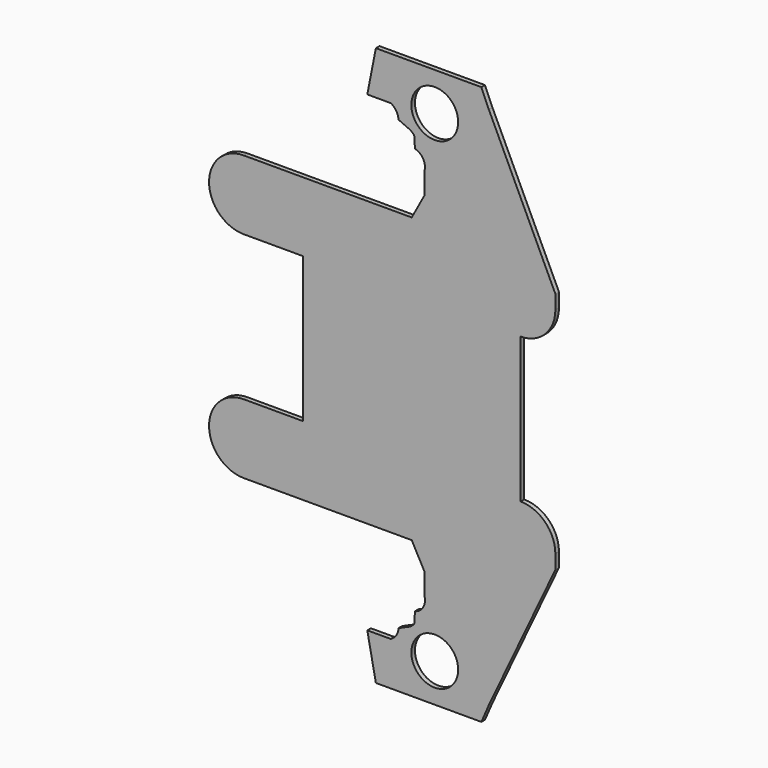
from build123d import *

# Parameters (mm, degrees)
F0_R     = 16.51
F1_DEPTH = 3.175


# Not quite as in the source:
# - ends of sketch curves that miss each other by under 0.0002 mm in the source are joined
# - a feature names something its author has since deleted; it is built from what else it names


with BuildPart() as f1:
    # F0 (on Front) → F1 (new body)
    with BuildSketch(Plane.XZ):
        with BuildLine():
            Line((72.172606051, -154.628444229), (72.172606051, -76.840944229))
            Line((72.172606051, -76.840944229), (72.172606051, -64.494198626))
            ThreePointArc((72.172606051, -64.494198626), (89.5045003647, -57.3150929397), (96.683606051, -39.983198626))
            Line((96.683606051, -39.983198626), (96.683606051, -30.0584486086))
            Line((96.683606051, -30.0584486086), (49.8026024117, 69.0988139849))
            Line((49.8026024117, 69.0988139849), (44.4719158113, 81.3992435336))
            Line((44.4719158113, 81.3992435336), (-29.9480052508, 81.3992435336))
            Line((-29.9480052508, 81.3992435336), (-35.9978974571, 50.6829957967))
            Line((-35.9978974571, 50.6829957967), (-19.4879078689, 50.6714224456))
            ThreePointArc((-19.4879078689, 50.6714224456), (-15.5812211009, 47.1637298884), (-13.9720730804, 42.1660573792))
            Line((-13.9720730804, 42.1660573792), (-5.4024819992, 38.3506346508))
            Line((-5.4024819992, 38.3506346508), (-2.9009456417, 36.1038269705))
            Line((-2.9009456417, 36.1038269705), (-2.3647786124, 27.9011076368))
            ThreePointArc((-2.3647786124, 27.9011076368), (3.4353485173, 23.5426794776), (4.3712937617, 16.3481414632))
            Line((4.3712937617, 16.3481414632), (4.2880811809, 16.2515226396))
            Line((4.2880811809, 16.2515226396), (4.2880776677, 1.0115236557))
            Line((4.2880776677, 1.0115236557), (-4.6405893252, -15.5276898319))
            Line((-4.6405893252, -15.5276898319), (-123.1544493252, -15.5276898319))
            ThreePointArc((-123.1544493252, -15.5276898319), (-147.6377037222, -40.010944229), (-123.1544493252, -64.494198626))
            Line((-123.1544493252, -64.494198626), (-81.4537847014, -64.494198626))
            Line((-81.4537847014, -64.494198626), (-81.4537847014, -76.840944229))
            Line((-81.4537847014, -76.840944229), (-81.4537847014, -154.628444229))
            Line((-81.4537847014, -154.628444229), (-81.4537847014, -166.9751898319))
            Line((-81.4537847014, -166.9751898319), (-123.1544493252, -166.9751898319))
            ThreePointArc((-123.1544493252, -166.9751898319), (-147.6377037222, -191.458444229), (-123.1544493252, -215.941698626))
            Line((-123.1544493252, -215.941698626), (-4.6405893252, -215.941698626))
            Line((-4.6405893252, -215.941698626), (4.2880776677, -232.4809121137))
            Line((4.2880776677, -232.4809121137), (4.2880811809, -247.7209110976))
            Line((4.2880811809, -247.7209110976), (4.3712937617, -247.8175299212))
            ThreePointArc((4.3712937617, -247.8175299212), (3.4353485173, -255.0120679356), (-2.3647786124, -259.3704960948))
            Line((-2.3647786124, -259.3704960948), (-2.9009456417, -267.5732154285))
            Line((-2.9009456417, -267.5732154285), (-5.4024819992, -269.8200231088))
            Line((-5.4024819992, -269.8200231088), (-13.9720735102, -273.6354510709))
            ThreePointArc((-13.9720735102, -273.6354510709), (-15.5812211009, -278.6331183464), (-19.487905219, -282.1408109018))
            Line((-19.487905219, -282.1408109018), (-35.9978974571, -282.1523842547))
            Line((-35.9978974571, -282.1523842547), (-29.9480052508, -312.8686319916))
            Line((-29.9480052508, -312.8686319916), (44.4719158113, -312.8686319916))
            Line((44.4719158113, -312.8686319916), (49.8026024117, -300.5682024429))
            Line((49.8026024117, -300.5682024429), (96.683606051, -201.4109398494))
            Line((96.683606051, -201.4109398494), (96.683606051, -191.4861898319))
            ThreePointArc((96.683606051, -191.4861898319), (89.5045003647, -174.1542955183), (72.172606051, -166.9751898319))
            Line((72.172606051, -166.9751898319), (72.172606051, -154.628444229))
        make_face()
        with Locations((11.6086210255, -285.7798588113)):
            Circle(F0_R, mode=Mode.SUBTRACT)
        with Locations((11.6086210255, 54.3104703533)):
            Circle(F0_R, mode=Mode.SUBTRACT)
    extrude(amount=F1_DEPTH)


solid = f1.part
